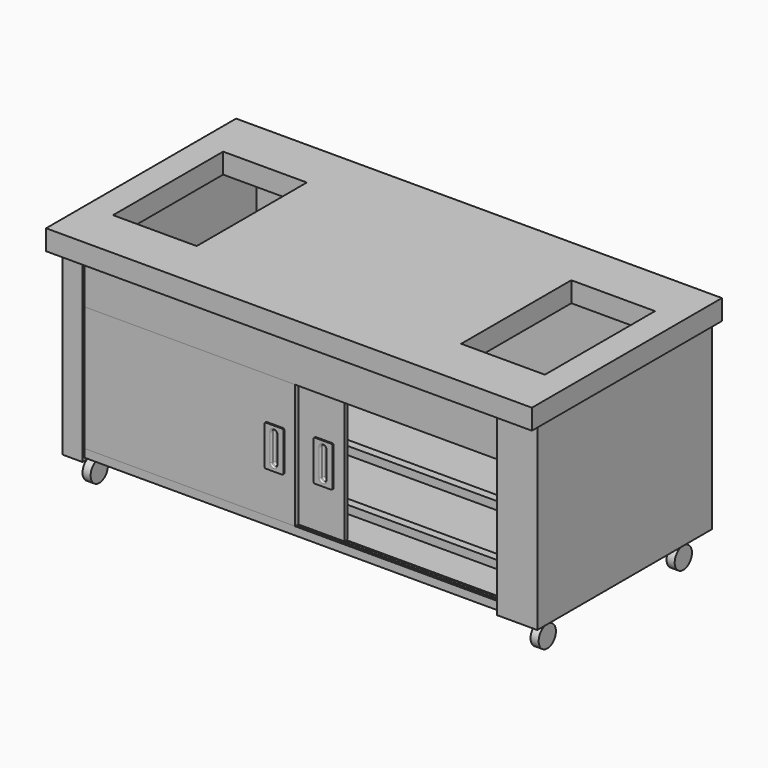
from build123d import *

# Parameters (mm, degrees)
F0_W           = 1800
F0_H           = 880
F1_DEPTH       = 75
F2_W           = 310
F2_H           = 510
F3_DEPTH       = 75.001
F4_W           = 75
F4_H           = 810
F4_W_2         = 150
F5_DEPTH       = 677
F6_W           = 30
F6_H           = 175
F7_DEPTH       = 1535
F8_W           = 800
F8_H           = 30
F9_DEPTH       = 1535
F10_W          = 1535
F10_H          = 5
F11_DEPTH      = 637
F12_W          = 700
F12_H          = 30
F13_DEPTH      = 1535
F14_W          = 1475
F14_H          = 640
F15_DEPTH      = 222
F16_W          = 5
F16_H          = 5
F17_DEPTH      = 1535
F18_W          = 15
F18_H          = 462
F19_DEPTH      = 780
F21_W          = 15
F21_H          = 462
F22_DEPTH      = 250
F23_W          = 70
F23_H          = 150
F24_DEPTH      = 5
F25_R          = 5
F26_DEPTH      = 10
F27_R          = 5
F28_W          = 70
F28_H          = 150
F29_DEPTH      = 5
F30_R          = 5
F31_DEPTH      = 10
F32_R          = 5
F33_R          = 4.99999
F33_2_R        = 4.99999
F35_R          = 40
F36_DEPTH      = 15
F36_DEPTH_BACK = 15
F38_R          = 40
F39_DEPTH      = 15
F39_DEPTH_BACK = 15


# Not quite as in the source:
# - a fillet or chamfer is up to 0.001 mm smaller than in the source, because OpenCascade refuses the exact size


with BuildPart() as f1:
    # F0 (on Top) → F1 (new body)
    with BuildSketch(Plane.XY):
        Rectangle(F0_W, F0_H)
    extrude(amount=F1_DEPTH)

    # F2 (on face) → F3 (cut, through all)
    with BuildSketch(Plane.XY.offset(75)):
        with Locations((-645, 0)):
            Rectangle(F2_W, F2_H)
        with Locations((645, 0)):
            Rectangle(F2_W, F2_H)
    extrude(amount=-F3_DEPTH, mode=Mode.SUBTRACT)

    # F4 (on face) → F5 (join)
    with BuildSketch(Plane(origin=(0, 0, 0), x_dir=(1, 0, 0), z_dir=(0, 0, -1))):
        with Locations((-842.5, -15)):
            Rectangle(F4_W, F4_H)
        with Locations((805, -15)):
            Rectangle(F4_W_2, F4_H)
    extrude(amount=F5_DEPTH)

    # F6 (on face) → F7 (join, through all)
    with BuildSketch(Plane(origin=(730, 0, 0), x_dir=(0, -1, 0), z_dir=(-1, 0, 0))):
        with Locations((365, -87.5)):
            Rectangle(F6_W, F6_H)
    extrude(amount=F7_DEPTH)


with BuildPart() as f9:
    # F8 (on face) → F9 (new body, through all)
    with BuildSketch(Plane.YZ.offset(-805)):
        with Locations((20, -652)):
            Rectangle(F8_W, F8_H)
    extrude(amount=F9_DEPTH)


with BuildPart() as f11:
    # F10 (on face) → F11 (new body, through all)
    with BuildSketch(Plane.XY.offset(-637)):
        with Locations((-37.5, 417.5)):
            Rectangle(F10_W, F10_H)
    extrude(amount=F11_DEPTH)


with BuildPart() as f13:
    # F12 (on face) → F13 (new body, through all)
    with BuildSketch(Plane.YZ.offset(-805)):
        with Locations((65, -390)):
            Rectangle(F12_W, F12_H)
    extrude(amount=F13_DEPTH)


with BuildPart() as f13b:
    # F12 (on face) → F13, piece 2 (new body, through all)
    with BuildSketch(Plane.YZ.offset(-805)):
        with Locations((65, -582)):
            Rectangle(F12_W, F12_H)
    extrude(amount=F13_DEPTH)


with BuildPart() as f15_tool:
    # F14 (on face) → F15 (new body, through all)
    with BuildSketch(Plane.XY.offset(-375)):
        with Locations((-37.5, 65)):
            Rectangle(F14_W, F14_H)
    extrude(amount=-F15_DEPTH)


with BuildPart() as f13_1:
    add(f13.part)

    # F15: cut by f15_tool
    add(f15_tool.part, mode=Mode.SUBTRACT)


with BuildPart() as f13b_1:
    add(f13b.part)

    # F15: cut by f15_tool
    add(f15_tool.part, mode=Mode.SUBTRACT)


with BuildPart() as f17_tool:
    # F16 (on face) → F17 (new body, through all)
    with BuildSketch(Plane.YZ.offset(-805)):
        with Locations((-372.5, -172.5)):
            Rectangle(F16_W, F16_H)
        with Locations((-372.5, -639.5)):
            Rectangle(F16_W, F16_H)
        with Locations((-357.5, -172.5)):
            Rectangle(F16_W, F16_H)
        with Locations((-357.5, -639.5)):
            Rectangle(F16_W, F16_H)
    extrude(amount=F17_DEPTH)


with BuildPart() as f1_1:
    add(f1.part)

    # F17: cut by f17_tool
    add(f17_tool.part, mode=Mode.SUBTRACT)


with BuildPart() as f9_1:
    add(f9.part)

    # F17: cut by f17_tool
    add(f17_tool.part, mode=Mode.SUBTRACT)


with BuildPart() as f19:
    # F18 (on face) → F19 (new body)
    with BuildSketch(Plane.YZ.offset(-805)):
        with Locations((-372.5, -406)):
            Rectangle(F18_W, F18_H)
    extrude(amount=F19_DEPTH)

    # F23 (on face) → F26 (cut)
    with BuildSketch(Plane.XZ.offset(380)):
        with BuildLine():
            ThreePointArc((-90, -356), (-100, -346), (-110, -356))
            Line((-110, -356), (-110, -456))
            ThreePointArc((-110, -456), (-100, -466), (-90, -456))
            Line((-90, -456), (-90, -356))
        make_face()
    extrude(amount=-F26_DEPTH, mode=Mode.SUBTRACT)

    # F27
    f27_edges = [f19.edges().sort_by_distance(p)[0] for p in [
        (-110, -370, -406),
    ]]
    fillet(f27_edges, radius=F27_R)


with BuildPart() as f22:
    # F21 (on offset) → F22 (new body)
    with BuildSketch(Plane.YZ.offset(-105)):
        with Locations((-357.5, -406)):
            Rectangle(F21_W, F21_H)
    extrude(amount=F22_DEPTH)

    # F28 (on face) → F31 (cut)
    with BuildSketch(Plane.XZ.offset(365)):
        with BuildLine():
            ThreePointArc((80, -356), (70, -346), (60, -356))
            Line((60, -356), (60, -456))
            ThreePointArc((60, -456), (70, -466), (80, -456))
            Line((80, -456), (80, -356))
        make_face()
    extrude(amount=-F31_DEPTH, mode=Mode.SUBTRACT)

    # F32
    f32_edges = [f22.edges().sort_by_distance(p)[0] for p in [
        (60, -355, -406),
    ]]
    fillet(f32_edges, radius=F32_R)


with BuildPart() as f24:
    # F23 (on face) → F24 (new body)
    with BuildSketch(Plane.XZ.offset(380)):
        with Locations((-100, -406)):
            Rectangle(F23_W, F23_H)
        with BuildLine():
            Line((-110, -456), (-110, -356))
            ThreePointArc((-110, -356), (-100, -346), (-90, -356))
            Line((-90, -356), (-90, -456))
            ThreePointArc((-90, -456), (-100, -466), (-110, -456))
        make_face(mode=Mode.SUBTRACT)
    extrude(amount=F24_DEPTH)

    # F25
    f25_edges = [f24.edges().sort_by_distance(p)[0] for p in [
        (-135, -382.5, -331),
        (-65, -382.5, -331),
        (-135, -382.5, -481),
        (-65, -382.5, -481),
    ]]
    fillet(f25_edges, radius=F25_R)

    # F33 (radius 5 in the source; OpenCascade refuses exactly that, so slightly less here)
    f33_edges = [f24.edges().sort_by_distance(p)[0] for p in [
        (-110, -385, -406),
    ]]
    fillet(f33_edges, radius=F33_R)


with BuildPart() as f29:
    # F28 (on face) → F29 (new body)
    with BuildSketch(Plane.XZ.offset(365)):
        with Locations((70, -406)):
            Rectangle(F28_W, F28_H)
        with BuildLine():
            Line((60, -456), (60, -356))
            ThreePointArc((60, -356), (70, -346), (80, -356))
            Line((80, -356), (80, -456))
            ThreePointArc((80, -456), (70, -466), (60, -456))
        make_face(mode=Mode.SUBTRACT)
    extrude(amount=F29_DEPTH)

    # F30
    f30_edges = [f29.edges().sort_by_distance(p)[0] for p in [
        (35, -367.5, -331),
        (105, -367.5, -331),
        (35, -367.5, -481),
        (105, -367.5, -481),
    ]]
    fillet(f30_edges, radius=F30_R)

    # F33#2 (radius 5 in the source; OpenCascade refuses exactly that, so slightly less here)
    f33_2_edges = [f29.edges().sort_by_distance(p)[0] for p in [
        (60, -370, -406),
    ]]
    fillet(f33_2_edges, radius=F33_2_R)


with BuildPart() as f36:
    # F35 (on offset) → F36 (new body, two sides)
    with BuildSketch(Plane.YZ.offset(830)) as f36_sk:
        with Locations((-300, -745)):
            Circle(F35_R)
    extrude(amount=F36_DEPTH)
    extrude(f36_sk.sketch, amount=-F36_DEPTH_BACK)


with BuildPart() as f36b:
    # F35 (on offset) → F36, piece 2 (new body, two sides)
    with BuildSketch(Plane.YZ.offset(830)) as f36_2_sk:
        with Locations((330, -745)):
            Circle(F35_R)
    extrude(amount=F36_DEPTH)
    extrude(f36_2_sk.sketch, amount=-F36_DEPTH_BACK)


with BuildPart() as f39:
    # F38 (on offset) → F39 (new body, two sides)
    with BuildSketch(Plane(origin=(-830, 0, 0), x_dir=(0, -1, 0), z_dir=(-1, 0, 0))) as f39_sk:
        with Locations((-330, -745)):
            Circle(F38_R)
    extrude(amount=F39_DEPTH)
    extrude(f39_sk.sketch, amount=-F39_DEPTH_BACK)


with BuildPart() as f39b:
    # F38 (on offset) → F39, piece 2 (new body, two sides)
    with BuildSketch(Plane(origin=(-830, 0, 0), x_dir=(0, -1, 0), z_dir=(-1, 0, 0))) as f39_2_sk:
        with Locations((300, -745)):
            Circle(F38_R)
    extrude(amount=F39_DEPTH)
    extrude(f39_2_sk.sketch, amount=-F39_DEPTH_BACK)


solid = Compound([f11.part, f13_1.part, f13b_1.part, f1_1.part, f9_1.part, f19.part, f22.part, f24.part, f29.part, f36.part, f36b.part, f39.part, f39b.part])
